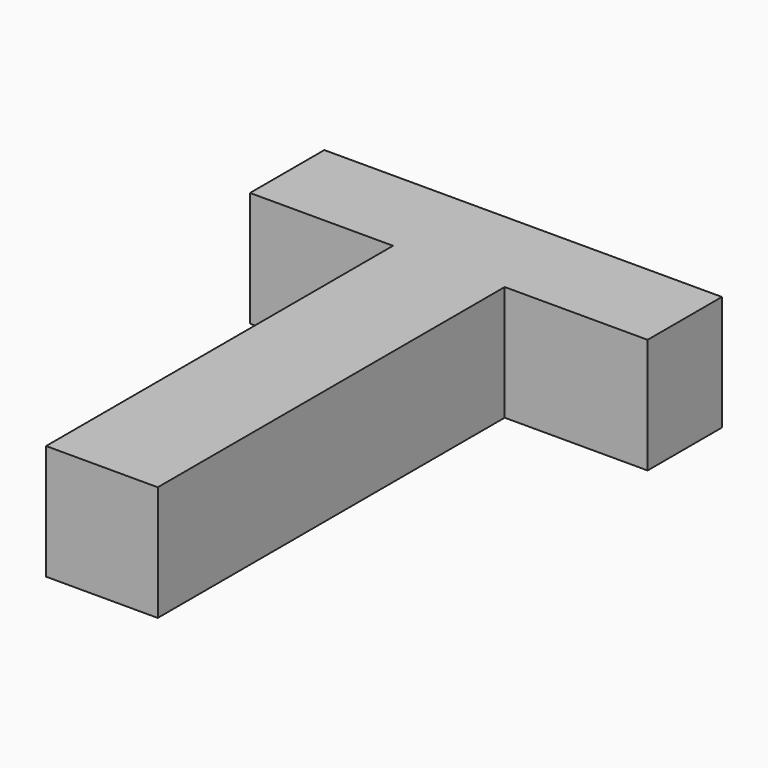
from build123d import *

# Parameters (mm, degrees)
F0_TEXT_SIZE = 40.7112446782
F1_DEPTH     = 6.35


# Not quite as in the source:
# - Text() gives the source's letters only with a copy of the font that has no kerning and outlines rounded to 1/6400 em; it was checked with that copy


with BuildPart() as f1:
    # F0 (on Top) → F1 (new body)
    with BuildSketch(Plane.XY):
        with Locations((-12.7, -14.6560480841)):
            Text('T', F0_TEXT_SIZE, font='Open Sans', font_style=FontStyle.BOLD, text_align=(TextAlign.LEFT, TextAlign.BOTTOM))
    extrude(amount=F1_DEPTH)


solid = f1.part
